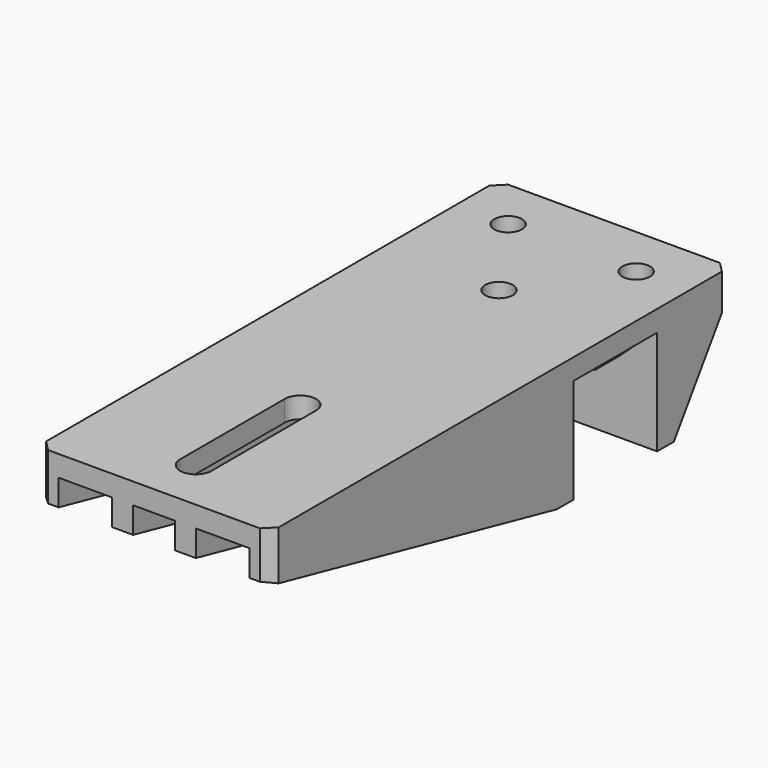
from build123d import *

# Parameters (mm, degrees)
F0_W      = 44.5
F0_H      = 110
F0_R      = 2.65
F1_DEPTH  = 4
F2_W      = 44.5
F2_H      = 4
F3_DEPTH  = 20
F4_W      = 4
F4_H      = 68.5
F4_H_2    = 13.5
F5_DEPTH  = 20
F7_DEPTH  = 20
F9_DEPTH  = 15
F11_DEPTH = 44.501
F12_DEPTH = 20.001
F14_DEPTH = 20
F15_W     = 44.5
F15_H     = 9
F16_DEPTH = 1.5
F17_SIZE  = 1.49999
F18_DEPTH = 20.001
F19_SIZE  = 2


# Not quite as in the source:
# - a fillet or chamfer is up to 0.001 mm smaller than in the source, because OpenCascade refuses the exact size


with BuildPart() as f1:
    # F0 (on Top) → F1 (new body)
    with BuildSketch(Plane.XY):
        with Locations((22.25, 55)):
            Rectangle(F0_W, F0_H)
        with BuildLine():
            Line((25.25, 35), (25.25, 10))
            ThreePointArc((25.25, 10), (22.25, 7), (19.25, 10))
            Line((19.25, 10), (19.25, 35))
            ThreePointArc((19.25, 35), (22.25, 38), (25.25, 35))
        make_face(mode=Mode.SUBTRACT)
        with Locations((10, 100)):
            Circle(F0_R, mode=Mode.SUBTRACT)
        with Locations((22.25, 82.5)):
            Circle(F0_R, mode=Mode.SUBTRACT)
        with Locations((34.5, 100)):
            Circle(F0_R, mode=Mode.SUBTRACT)
    extrude(amount=F1_DEPTH)

    # F2 (on face) → F3 (join)
    with BuildSketch(Plane(origin=(0, 0, 0), x_dir=(1, 0, 0), z_dir=(0, 0, -1))):
        with Locations((22.25, -94.5)):
            Rectangle(F2_W, F2_H)
        with Locations((22.25, -70.5)):
            Rectangle(F2_W, F2_H)
    extrude(amount=F3_DEPTH)

    # F4 (on face) → F5 (join)
    with BuildSketch(Plane(origin=(0, 0, 0), x_dir=(1, 0, 0), z_dir=(0, 0, -1))):
        with Locations((2, -34.25)):
            Rectangle(F4_W, F4_H)
        with Locations((42.5, -34.25)):
            Rectangle(F4_W, F4_H)
        Polygon((0, -96.5), (0, -110), (4, -110), (4, -103.4641016151), (4, -96.5358983849), (4, -96.5), align=None)
        Polygon((4, -96.5358983849), (4, -103.4641016151), (10, -106.9282032303), (16, -103.4641016151), (16, -96.5358983849), (15.9378221735, -96.5), (11.9378221735, -96.5), (14, -97.6905989232), (14, -102.3094010768), (10, -104.6188021535), (6, -102.3094010768), (6, -97.6905989232), (8.0621778265, -96.5), (4.0621778265, -96.5), align=None)
        Polygon((11.9378221735, -96.5), (8.0621778265, -96.5), (6, -97.6905989232), (6, -102.3094010768), (10, -104.6188021535), (14, -102.3094010768), (14, -97.6905989232), align=None)
        Polygon((40.5, -110), (44.5, -110), (44.5, -96.5), (40.5, -96.5), (40.5, -96.5358983849), (40.5, -103.4641016151), align=None)
        Polygon((34.5, -106.9282032303), (40.5, -103.4641016151), (40.5, -96.5358983849), (40.4378221735, -96.5), (36.4378221735, -96.5), (38.5, -97.6905989232), (38.5, -102.3094010768), (34.5, -104.6188021535), (30.5, -102.3094010768), (30.5, -97.6905989232), (32.5621778265, -96.5), (28.5621778265, -96.5), (28.5, -96.5358983849), (28.5, -103.4641016151), align=None)
        Polygon((38.5, -97.6905989232), (36.4378221735, -96.5), (32.5621778265, -96.5), (30.5, -97.6905989232), (30.5, -102.3094010768), (34.5, -104.6188021535), (38.5, -102.3094010768), align=None)
        Polygon((32.5621778265, -96.5), (36.4378221735, -96.5), (34.5, -95.3811978465), align=None)
        with Locations((16.25, -34.25)):
            Rectangle(F4_W, F4_H)
        with Locations((28.25, -34.25)):
            Rectangle(F4_W, F4_H)
        with Locations((22.25, -103.25)):
            Rectangle(F4_W, F4_H_2)
    extrude(amount=F5_DEPTH)

    # F6 (on face) → F7 (join)
    with BuildSketch(Plane(origin=(0, 0, 0), x_dir=(1, 0, 0), z_dir=(0, 0, -1))):
        Polygon((40.5, -96.5), (40.4378221735, -96.5), (40.5, -96.5358983849), align=None)
        Polygon((4.0621778265, -96.5), (4, -96.5), (4, -96.5358983849), align=None)
        Polygon((16, -96.5358983849), (16, -103.4641016151), (20.25, -103.4641016151), (20.25, -96.5), (15.9378221735, -96.5), align=None)
        Polygon((28.5621778265, -96.5), (24.25, -96.5), (24.25, -103.4641016151), (28.5, -103.4641016151), (28.5, -96.5358983849), align=None)
    extrude(amount=F7_DEPTH)

    # F8 (on face) → F9 (cut)
    with BuildSketch(Plane(origin=(0, 0, -20), x_dir=(1, 0, 0), z_dir=(0, 0, -1))):
        Polygon((4, -103.4641016151), (10, -106.9282032303), (16, -103.4641016151), (20.25, -103.4641016151), (20.25, -96.5), (4, -96.5), align=None)
        Polygon((24.25, -103.4641016151), (28.5, -103.4641016151), (34.5, -106.9282032303), (40.5, -103.4641016151), (40.5, -96.5), (24.25, -96.5), align=None)
    extrude(amount=-F9_DEPTH, mode=Mode.SUBTRACT)

    # F10 (on face) → F11 (cut, through all)
    with BuildSketch(Plane(origin=(0, 0, 0), x_dir=(0, -1, 0), z_dir=(-1, 0, 0))):
        Polygon((-96.5, -20), (-110, 0), (-110, -20), align=None)
        Polygon((0, -5), (-68.5, -20), (0, -20), align=None)
    extrude(amount=-F11_DEPTH, mode=Mode.SUBTRACT)

    # F12 (cut, through all): faces of the model
    f12_faces = [f1.faces().sort_by_distance(p)[0] for p in [
        (34.5, 100, 0),
        (10, 100, 0),
    ]]
    extrude(f12_faces, amount=-F12_DEPTH, mode=Mode.SUBTRACT)

    # F13 (on face) → F14 (cut, through all)
    with BuildSketch(Plane(origin=(0, 0, -20), x_dir=(1, 0, 0), z_dir=(0, 0, -1))):
        Polygon((14, -102.3094010768), (14, -97.6905989232), (10, -95.3811978465), (6, -97.6905989232), (6, -102.3094010768), (10, -104.6188021535), align=None)
        Polygon((38.5, -102.3094010768), (38.5, -97.6905989232), (34.5, -95.3811978465), (30.5, -97.6905989232), (30.5, -102.3094010768), (34.5, -104.6188021535), align=None)
    extrude(amount=-F14_DEPTH, mode=Mode.SUBTRACT)

    # F15 (on face) → F16 (join)
    with BuildSketch(Plane(origin=(0, 0, 0), x_dir=(1, 0, 0), z_dir=(0, 0, -1))):
        with Locations((22.25, -82.5)):
            Rectangle(F15_W, F15_H)
    extrude(amount=F16_DEPTH)

    # F17 (size 1.5 in the source; OpenCascade refuses exactly that, so slightly less here)
    f17_edges = [f1.edges().sort_by_distance(p)[0] for p in [
        (44.5, 82.5, -1.5),
        (22.25, 78, -1.5),
        (0, 82.5, -1.5),
        (22.25, 87, -1.5),
    ]]
    chamfer(f17_edges, length=F17_SIZE)

    # F18 (cut, through all): a face of the model
    f18_faces = [f1.faces().sort_by_distance(p)[0] for p in [
        (22.25, 82.5, 0),
    ]]
    extrude(f18_faces, amount=-F18_DEPTH, mode=Mode.SUBTRACT)

    # F19
    f19_edges = [f1.edges().sort_by_distance(p)[0] for p in [
        (44.5, 110, 2),
        (0, 110, 2),
        (0, 0, -0.5),
        (44.5, 0, -0.5),
    ]]
    chamfer(f19_edges, length=F19_SIZE)


solid = f1.part
